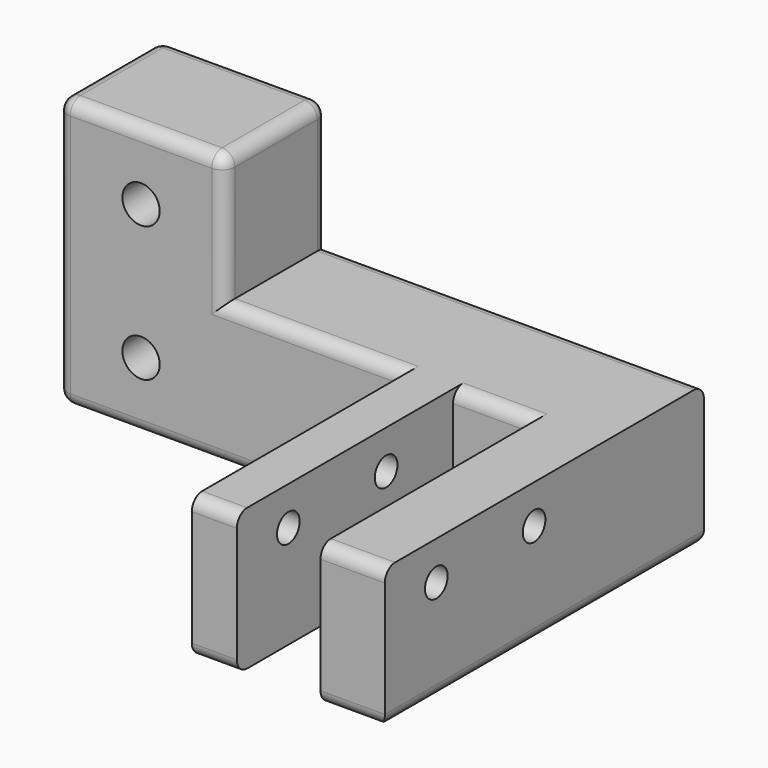
from build123d import *

# Parameters (mm, degrees)
F0_W          = 16.5
F0_H          = 11
F1_DEPTH      = 10
F2_W          = 5
F2_H          = 11
F3_DEPTH      = 21
F4_R          = 1.1
F5_DEPTH      = 25
F6_W          = 1.5
F6_H          = 11
F7_DEPTH      = 21
F8_DEPTH      = 25.75
F9_W          = 13
F9_H          = 10
F10_DEPTH     = 10
F11_R         = 3
F12_DEPTH     = 3.5
F13_R         = 1.45
F14_DEPTH     = 25
F15_R         = 1
F16_T1_DEPTH  = 11
F16_S5_W      = 1
F16_S5_H      = 1
F16_T6_DEPTH  = 1
F16_S11_W     = 1
F16_S11_H     = 1
F16_T12_DEPTH = 1


# Not quite as in the source:
# - a fillet or chamfer that OpenCascade refuses, or shapes differently, is made with other operations: its cross-section is extruded or revolved along the edge and cut away or added


with BuildPart() as f1:
    # F0 (on Front) → F1 (new body)
    with BuildSketch(Plane.XZ):
        with Locations((8.25, 5.5)):
            Rectangle(F0_W, F0_H)
    extrude(amount=F1_DEPTH)

    # F2 (on face) → F3 (join)
    with BuildSketch(Plane.XZ.offset(10)):
        with Locations((14, 5.5)):
            Rectangle(F2_W, F2_H)
        with Locations((2.5, 5.5)):
            Rectangle(F2_W, F2_H)
    extrude(amount=F3_DEPTH)

    # F4 (on face) → F5 (cut)
    with BuildSketch(Plane(origin=(0, 0, 0), x_dir=(0, -1, 0), z_dir=(-1, 0, 0))):
        with BuildLine():
            ThreePointArc((24.9, 8), (26, 6.9), (27.1, 8))
            Line((27.1, 8), (26, 8))
            Line((26, 8), (24.9, 8))
        make_face()
        with BuildLine():
            Line((26, 8), (27.1, 8))
            ThreePointArc((27.1, 8), (26, 9.1), (24.9, 8))
            Line((24.9, 8), (26, 8))
        make_face()
        with Locations((16.5, 8)):
            Circle(F4_R)
    extrude(amount=-F5_DEPTH, mode=Mode.SUBTRACT)

    # F6 (on face) → F7 (cut)
    with BuildSketch(Plane.XZ.offset(31)):
        with Locations((0.75, 5.5)):
            Rectangle(F6_W, F6_H)
    extrude(amount=-F7_DEPTH, mode=Mode.SUBTRACT)

    # F8 (add): a face of the model
    f8_faces = [f1.faces().sort_by_distance(p)[0] for p in [
        (0, -5, 5.5),
    ]]
    extrude(f8_faces, amount=F8_DEPTH)

    # F9 (on face) → F10 (join)
    with BuildSketch(Plane.XY.offset(11)):
        with Locations((-19.25, -5)):
            Rectangle(F9_W, F9_H)
    extrude(amount=F10_DEPTH)

    # F11 (on face) → F12 (cut)
    with BuildSketch(Plane(origin=(0, 0, 0), x_dir=(-1, 0, 0), z_dir=(0, 1, 0))):
        with BuildLine():
            ThreePointArc((22.25, 15.75), (21.3713203436, 17.8713203436), (19.25, 18.75))
            Line((19.25, 18.75), (19.25, 12.75))
            ThreePointArc((19.25, 12.75), (21.3713203436, 13.6286796564), (22.25, 15.75))
        make_face()
        with BuildLine():
            Line((19.25, 12.75), (19.25, 18.75))
            ThreePointArc((19.25, 18.75), (16.25, 15.75), (19.25, 12.75))
        make_face()
        with Locations((19.25, 5.25)):
            Circle(F11_R)
    extrude(amount=-F12_DEPTH, mode=Mode.SUBTRACT)

    # F13 (on face) → F14 (cut)
    with BuildSketch(Plane(origin=(0, 0, 0), x_dir=(-1, 0, 0), z_dir=(0, 1, 0))):
        with Locations((19.25, 15.75)):
            Circle(F13_R)
        with Locations((19.25, 5.25)):
            Circle(F13_R)
    extrude(amount=-F14_DEPTH, mode=Mode.SUBTRACT)

    # F15
    f15_edges = [f1.edges().sort_by_distance(p)[0] for p in [
        (-12.75, -5, 21),
        (-25.75, -5, 21),
        (-19.25, 0, 21),
        (-25.75, 0, 10.5),
        (-25.75, -10, 10.5),
        (-25.75, -5, 0),
        (-4.625, 0, 0),
        (-12.125, -10, 0),
        (-12.75, 0, 16),
        (-12.75, -10, 16),
        (1.875, 0, 11),
        (-5.625, -10, 11),
        (8.25, -10, 11),
        (8.25, -10, 0),
        (3.25, -31, 11),
        (14, -31, 11),
        (14, -31, 0),
        (16.5, -15.5, 0),
        (3.25, -31, 0),
    ]]
    fillet(f15_edges, radius=F15_R)

    # F16: fillet of radius 1 on 1 edges, made by hand

    # F16_s2 → F16_t1 (cut)
    with BuildSketch(Plane.YZ.offset(-24.75)):
        with BuildLine():
            ThreePointArc((-10, 20), (-9.7071067812, 20.7071067812), (-9, 21))
            Line((-9, 21), (-10, 21))
            Line((-10, 21), (-10, 20))
        make_face()
    extrude(amount=F16_T1_DEPTH, mode=Mode.SUBTRACT)


with BuildPart() as f16_tool4:
    # F16_s5 → F16_t6 (new body)
    with BuildSketch(Plane.XZ.offset(9)):
        with Locations((-25.25, 20.5)):
            Rectangle(F16_S5_W, F16_S5_H)
    extrude(amount=F16_T6_DEPTH)

    # F16_s7 → F16_t8 (revolve, cut)
    with BuildSketch(Plane(origin=(-24.75, -9, 20), x_dir=(0.7071067812, 0, -0.7071067812), z_dir=(-0.7071067812, 0, -0.7071067812))):
        with BuildLine():
            ThreePointArc((0, -1), (1, 0), (0, 1))
            Line((0, 1), (0, -1))
        make_face()
    revolve(axis=Axis((-24.75, -9, 20), (0, -1, 0)), mode=Mode.SUBTRACT)


with BuildPart() as f1_1:
    add(f1.part)

    # F16_t3: cut F16_tool4
    add(f16_tool4.part, mode=Mode.SUBTRACT)


with BuildPart() as f16_tool10:
    # F16_s11 → F16_t12 (new body)
    with BuildSketch(Plane.XZ.offset(9)):
        with Locations((-13.25, 20.5)):
            Rectangle(F16_S11_W, F16_S11_H)
    extrude(amount=F16_T12_DEPTH)

    # F16_s13 → F16_t14 (revolve, cut)
    with BuildSketch(Plane(origin=(-13.75, -9, 20), x_dir=(-0.7071067812, 0, -0.7071067812), z_dir=(-0.7071067812, 0, 0.7071067812))):
        with BuildLine():
            ThreePointArc((0, -1), (1, 0), (0, 1))
            Line((0, 1), (0, -1))
        make_face()
    revolve(axis=Axis((-13.75, -9, 20), (0, -1, 0)), mode=Mode.SUBTRACT)


with BuildPart() as f1_2:
    add(f1_1.part)

    # F16_t9: cut F16_tool10
    add(f16_tool10.part, mode=Mode.SUBTRACT)


solid = f1_2.part
